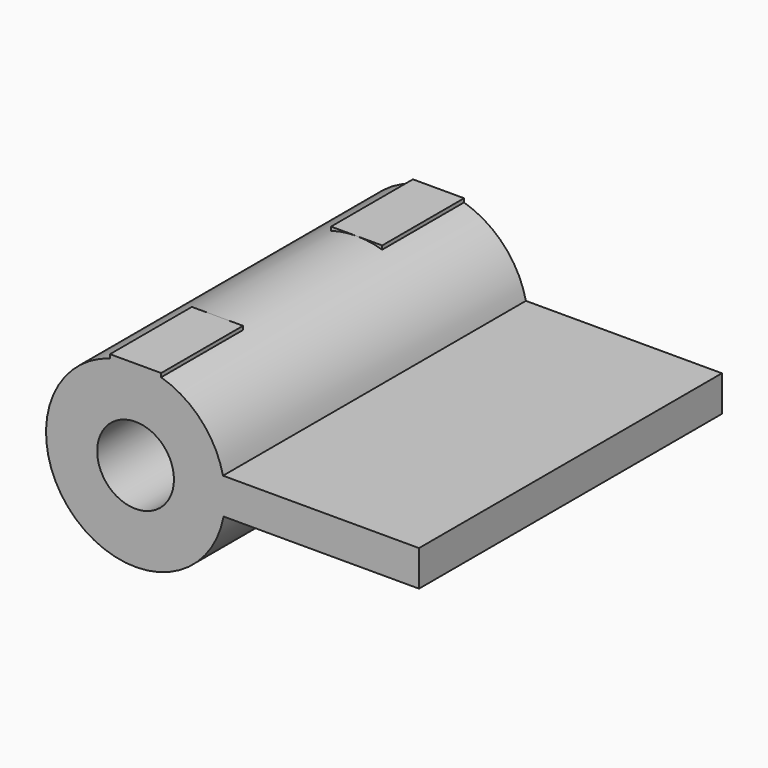
from build123d import *

# Parameters (mm, degrees)
F0_R     = 11.1125
F0_R_2   = 4.7625
F1_DEPTH = 46.99
F2_W     = 12.7
F2_H     = 3.7792036489
F2_H_2   = 3.4237923279
F3_DEPTH = 3.175
F5_W     = 46.99
F5_H     = 4.4356931467
F6_DEPTH = 25.4
F7_R     = 4.92125
F8_DEPTH = 25.4


# Not quite as in the source:
# - a feature names something its author has since deleted; it is built from what else it names


with BuildPart() as f1:
    # F0 (on Front) → F1 (new body)
    with BuildSketch(Plane.XZ):
        Circle(F0_R)
        Circle(F0_R_2, mode=Mode.SUBTRACT)
    extrude(amount=F1_DEPTH)

    # F2 (on Right) → F3 (join, symmetric)
    with BuildSketch(Plane.YZ):
        with Locations((-40.64, 9.2228981756)):
            Rectangle(F2_W, F2_H)
        with Locations((-6.35, 9.400603836)):
            Rectangle(F2_W, F2_H_2)
    extrude(amount=F3_DEPTH, both=True)

    # F5 (on offset) → F6 (join)
    with BuildSketch(Plane.YZ.offset(9.779)):
        with Locations((-23.495, 0.1773260301)):
            Rectangle(F5_W, F5_H)
    extrude(amount=F6_DEPTH)

    # F7 (on Right) → F8 (cut)
    with BuildSketch(Plane.YZ):
        with Locations((-23.495, 0)):
            Circle(F7_R)
    extrude(amount=-F8_DEPTH, mode=Mode.SUBTRACT)


solid = f1.part
